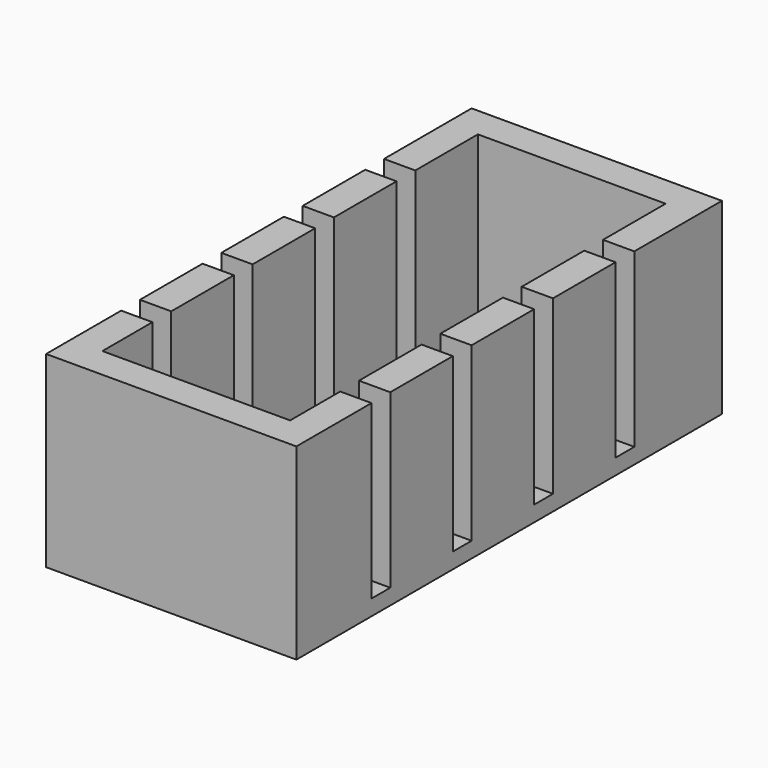
from build123d import *

# Parameters (mm, degrees)
F0_W     = 40.64
F0_H     = 86.36
F0_W_2   = 30.48
F0_H_2   = 76.2
F1_DEPTH = 30.48
F2_DEPTH = 2.54
F3_W     = 5.08
F3_H     = 3.81
F4_DEPTH = 27.94


# Not quite as in the source:
# - a feature names something its author has since deleted; it is built from what else it names


with BuildPart() as f1:
    # F0 (on Top) → F1 (new body)
    with BuildSketch(Plane.XY):
        Rectangle(F0_W, F0_H)
        Rectangle(F0_W_2, F0_H_2, mode=Mode.SUBTRACT)
    extrude(amount=F1_DEPTH)

    # F0 (on Top) → F2 (join)
    with BuildSketch(Plane.XY):
        Rectangle(F0_W_2, F0_H_2)
    extrude(amount=F2_DEPTH)

    # F3 (on face) → F4 (cut)
    with BuildSketch(Plane.XY.offset(30.48)):
        with Locations((-17.78, 23.495)):
            Rectangle(F3_W, F3_H)
        with Locations((17.78, 23.495)):
            Rectangle(F3_W, F3_H)
        with Locations((17.78, 6.985)):
            Rectangle(F3_W, F3_H)
        with Locations((-17.78, 6.985)):
            Rectangle(F3_W, F3_H)
        with Locations((-17.78, -9.525)):
            Rectangle(F3_W, F3_H)
        with Locations((17.78, -9.525)):
            Rectangle(F3_W, F3_H)
        with Locations((-17.78, -26.035)):
            Rectangle(F3_W, F3_H)
        with Locations((17.78, -26.035)):
            Rectangle(F3_W, F3_H)
    extrude(amount=-F4_DEPTH, mode=Mode.SUBTRACT)


solid = f1.part
